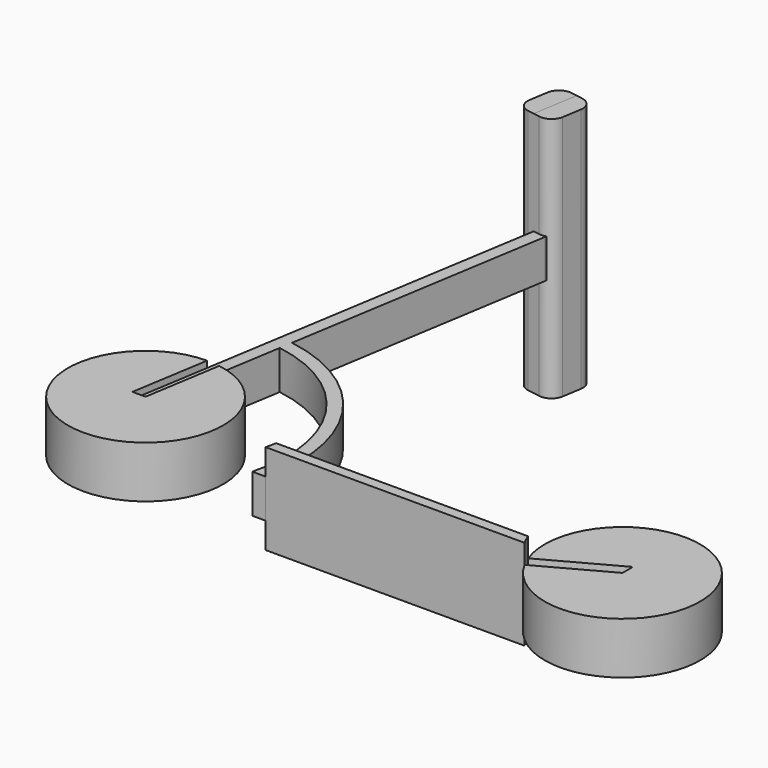
from build123d import *

# Parameters (mm, degrees)
F1_DEPTH      = 50.8
F1_DEPTH_BACK = 50.8
F2_DEPTH      = 38.1
F2_DEPTH_BACK = 38.1
F3_DEPTH      = 88.9
F3_DEPTH_BACK = 88.9
F6_DEPTH      = 88.9
F7_T1_DEPTH   = 609.6
F7_T6_DEPTH   = 609.6
F7_T12_DEPTH  = 609.6
F7_T18_DEPTH  = 609.6
F7_T25_DEPTH  = 609.6
F7_T31_DEPTH  = 609.6


# Not quite as in the source:
# - a fillet or chamfer that OpenCascade refuses, or shapes differently, is made with other operations: its cross-section is extruded or revolved along the edge and cut away or added


with BuildPart() as f1:
    # F0 (on Top) → F1 (new body, two sides)
    with BuildSketch(Plane.XY) as f1_sk:
        with BuildLine():
            ThreePointArc((-783.3901008351, 0), (-819.7667936825, 98.8147367419), (-911.5312057875, 150.4568576405))
            Line((-911.5312057875, 150.4568576405), (-935.7901008351, 0))
            Line((-935.7901008351, 0), (-961.5181404919, 0))
            Line((-961.5181404919, 0), (-936.9466506832, 152.3956114606))
            ThreePointArc((-936.9466506832, 152.3956114606), (-1043.1434934298, -108.1712027225), (-783.3901008351, 0))
        make_face()
    extrude(amount=F1_DEPTH)
    extrude(f1_sk.sketch, amount=-F1_DEPTH_BACK)


with BuildPart() as f1b:
    # F0 (on Top) → F1, piece 2 (new body, two sides)
    with BuildSketch(Plane.XY) as f1_2_sk:
        with BuildLine():
            ThreePointArc((-133.8252661358, -72.9147320071), (37.6217320235, -147.6833276966), (152.4, 0))
            ThreePointArc((152.4, 0), (-26.6841566333, 150.0457123172), (-143.0555877267, -52.5438751919))
            Line((-143.0555877267, -52.5438751919), (0, 25.4))
            Line((0, 25.4), (0, 0))
            Line((0, 0), (-133.8252661358, -72.9147320071))
        make_face()
    extrude(amount=F1_DEPTH)
    extrude(f1_2_sk.sketch, amount=-F1_DEPTH_BACK)


with BuildPart() as f2:
    # F0 (on Top) → F2 (new body, two sides)
    with BuildSketch(Plane.XY) as f2_sk:
        with BuildLine():
            Line((-891.6222432269, 273.9348618882), (-887.5790940523, 299.0110048283))
            Line((-887.5790940523, 299.0110048283), (-804.3877526602, 814.9746455529))
            Line((-804.3877526602, 814.9746455529), (-829.4638956003, 819.0177947275))
            Line((-829.4638956003, 819.0177947275), (-936.9466506832, 152.3956114606))
            ThreePointArc((-936.9466506832, 152.3956114606), (-924.1983244388, 151.9585164444), (-911.5312057875, 150.4568576405))
            Line((-911.5312057875, 150.4568576405), (-891.6222432269, 273.9348618882))
        make_face()
        with BuildLine():
            Line((-935.7901008351, 0), (-911.5312057875, 150.4568576405))
            ThreePointArc((-911.5312057875, 150.4568576405), (-924.1983244388, 151.9585164444), (-936.9466506832, 152.3956114606))
            Line((-936.9466506832, 152.3956114606), (-961.5181404919, 0))
            Line((-961.5181404919, 0), (-935.7901008351, 0))
        make_face()
        with BuildLine():
            ThreePointArc((-641.8252661358, -72.9147320071), (-639.4925118211, -62.7663996731), (-637.5099919387, -52.5438751919))
            ThreePointArc((-637.5099919387, -52.5438751919), (-688.9870787149, 175.5566873001), (-887.5790940523, 299.0110048283))
            Line((-887.5790940523, 299.0110048283), (-891.6222432269, 273.9348618882))
            ThreePointArc((-891.6222432269, 273.9348618882), (-702.5631088402, 150.3205854446), (-668.0690705447, -72.9147320071))
            Line((-668.0690705447, -72.9147320071), (-641.8252661358, -72.9147320071))
        make_face()
    extrude(amount=F2_DEPTH)
    extrude(f2_sk.sketch, amount=-F2_DEPTH_BACK)

    # F5 (on line) → F6 (join)
    with BuildSketch(Plane(origin=(107.6913114103, 667.9156770389, 0), x_dir=(0.9872497221, -0.1591791014, 0), z_dir=(-0.1591791014, -0.9872497221, 0))):
        Polygon((-911.0927623749, 0), (-911.0927623749, 241.3), (-949.192252238, 241.4971602735), (-987.291742101, 241.3), (-987.291742101, 0), (-987.291742101, -241.3), (-949.1927623749, -241.3), (-911.0927623749, -241.3), align=None)
    extrude(amount=-F6_DEPTH)

    # F7: fillet of radius 25.4 on 4 edges, made by hand

    # F7_s2 → F7_t1 (cut)
    with BuildSketch(Plane.XY.offset(-304.8)):
        with BuildLine():
            ThreePointArc((-781.6768920702, 875.6329615621), (-786.1625860927, 894.5486832569), (-802.7098858357, 904.7522536768))
            Line((-802.7098858357, 904.7522536768), (-777.6337428956, 900.7091045022))
            Line((-777.6337428956, 900.7091045022), (-781.6768920702, 875.6329615621))
        make_face()
        with BuildLine():
            ThreePointArc((-827.7850215107, 908.7952404451), (-846.7007432055, 904.3095464227), (-856.9043136254, 887.7622466796))
            Line((-856.9043136254, 887.7622466796), (-852.8611644508, 912.8383896197))
            Line((-852.8611644508, 912.8383896197), (-827.7850215107, 908.7952404451))
        make_face()
        with BuildLine():
            ThreePointArc((-841.9360436219, 821.0287401548), (-858.4833433649, 831.2323105747), (-862.9690373873, 850.1480322695))
            Line((-862.9690373873, 850.1480322695), (-867.0121865619, 825.0718893294))
            Line((-867.0121865619, 825.0718893294), (-841.9360436219, 821.0287401548))
        make_face()
    extrude(amount=F7_T1_DEPTH, mode=Mode.SUBTRACT)


with BuildPart() as f2b:
    # F0 (on Top) → F2, piece 2 (new body, two sides)
    with BuildSketch(Plane.XY) as f2_2_sk:
        with BuildLine():
            Line((0, 25.4), (-143.0555877267, -52.5438751919))
            ThreePointArc((-143.0555877267, -52.5438751919), (-138.8146057184, -62.8988492681), (-133.8252661358, -72.9147320071))
            Line((-133.8252661358, -72.9147320071), (0, 0))
            Line((0, 0), (0, 25.4))
        make_face()
    extrude(amount=F2_DEPTH)
    extrude(f2_2_sk.sketch, amount=-F2_DEPTH_BACK)


with BuildPart() as f3:
    # F0 (on Top) → F3 (new body, two sides)
    with BuildSketch(Plane.XY) as f3_sk:
        with BuildLine():
            ThreePointArc((-133.8252661358, -72.9147320071), (-138.8146057184, -62.8988492681), (-143.0555877267, -52.5438751919))
            Line((-143.0555877267, -52.5438751919), (-637.5099919387, -52.5438751919))
            ThreePointArc((-637.5099919387, -52.5438751919), (-639.4925118211, -62.7663996731), (-641.8252661358, -72.9147320071))
            Line((-641.8252661358, -72.9147320071), (-133.8252661358, -72.9147320071))
        make_face()
    extrude(amount=F3_DEPTH)
    extrude(f3_sk.sketch, amount=-F3_DEPTH_BACK)


with BuildPart() as f7_tool4:
    # F7_s5 → F7_t6 (new body)
    with BuildSketch(Plane.XY.offset(304.8)):
        with BuildLine():
            ThreePointArc((-787.7416158321, 838.0187471519), (-797.945186252, 821.4714474089), (-816.8609079468, 816.9857533865))
            Line((-816.8609079468, 816.9857533865), (-791.7847650068, 812.9426042119))
            Line((-791.7847650068, 812.9426042119), (-787.7416158321, 838.0187471519))
        make_face()
    extrude(amount=-F7_T6_DEPTH)

    split(bisect_by=Plane.XY.offset(38.1), keep=Keep.TOP)

    split(bisect_by=Plane(origin=(-912.0790640705, 147.058968514, 0), x_dir=(0, 0, 1), z_dir=(0.9872497221, -0.1591791014, 0)), keep=Keep.TOP)


with BuildPart() as f2_1:
    add(f2.part)

    # F7_t3: cut F7_tool4
    add(f7_tool4.part, mode=Mode.SUBTRACT)


with BuildPart() as f7_tool10:
    # F7_s11 → F7_t12 (new body)
    with BuildSketch(Plane.XY.offset(304.8)):
        with BuildLine():
            ThreePointArc((-787.7416158321, 838.0187471519), (-797.945186252, 821.4714474089), (-816.8609079468, 816.9857533865))
            Line((-816.8609079468, 816.9857533865), (-791.7847650068, 812.9426042119))
            Line((-791.7847650068, 812.9426042119), (-787.7416158321, 838.0187471519))
        make_face()
    extrude(amount=-F7_T12_DEPTH)

    split(bisect_by=Plane.XY.offset(38.1), keep=Keep.TOP)

    split(bisect_by=Plane(origin=(-912.0790640705, 147.058968514, 0), x_dir=(0, 0, 1), z_dir=(-0.9872497221, 0.1591791014, 0)), keep=Keep.TOP)


with BuildPart() as f2_2:
    add(f2_1.part)

    # F7_t9: cut F7_tool10
    add(f7_tool10.part, mode=Mode.SUBTRACT)


with BuildPart() as f7_tool16:
    # F7_s17 → F7_t18 (new body)
    with BuildSketch(Plane.XY.offset(304.8)):
        with BuildLine():
            ThreePointArc((-787.7416158321, 838.0187471519), (-797.945186252, 821.4714474089), (-816.8609079468, 816.9857533865))
            Line((-816.8609079468, 816.9857533865), (-791.7847650068, 812.9426042119))
            Line((-791.7847650068, 812.9426042119), (-787.7416158321, 838.0187471519))
        make_face()
    extrude(amount=-F7_T18_DEPTH)

    split(bisect_by=Plane.XY.offset(38.1), keep=Keep.BOTTOM)

    split(bisect_by=Plane.XY.offset(-38.1), keep=Keep.TOP)

    split(bisect_by=Plane(origin=(-912.0790640705, 147.058968514, 0), x_dir=(0, 0, 1), z_dir=(0.9872497221, -0.1591791014, 0)), keep=Keep.TOP)


with BuildPart() as f2_3:
    add(f2_2.part)

    # F7_t15: cut F7_tool16
    add(f7_tool16.part, mode=Mode.SUBTRACT)


with BuildPart() as f7_tool23:
    # F7_s24 → F7_t25 (new body)
    with BuildSketch(Plane.XY.offset(304.8)):
        with BuildLine():
            ThreePointArc((-787.7416158321, 838.0187471519), (-797.945186252, 821.4714474089), (-816.8609079468, 816.9857533865))
            Line((-816.8609079468, 816.9857533865), (-791.7847650068, 812.9426042119))
            Line((-791.7847650068, 812.9426042119), (-787.7416158321, 838.0187471519))
        make_face()
    extrude(amount=-F7_T25_DEPTH)

    split(bisect_by=Plane.XY.offset(-38.1), keep=Keep.BOTTOM)

    split(bisect_by=Plane(origin=(-912.0790640705, 147.058968514, 0), x_dir=(0, 0, 1), z_dir=(0.9872497221, -0.1591791014, 0)), keep=Keep.TOP)


with BuildPart() as f2_4:
    add(f2_3.part)

    # F7_t22: cut F7_tool23
    add(f7_tool23.part, mode=Mode.SUBTRACT)


with BuildPart() as f7_tool29:
    # F7_s30 → F7_t31 (new body)
    with BuildSketch(Plane.XY.offset(304.8)):
        with BuildLine():
            ThreePointArc((-787.7416158321, 838.0187471519), (-797.945186252, 821.4714474089), (-816.8609079468, 816.9857533865))
            Line((-816.8609079468, 816.9857533865), (-791.7847650068, 812.9426042119))
            Line((-791.7847650068, 812.9426042119), (-787.7416158321, 838.0187471519))
        make_face()
    extrude(amount=-F7_T31_DEPTH)

    split(bisect_by=Plane.XY.offset(-38.1), keep=Keep.BOTTOM)

    split(bisect_by=Plane(origin=(-912.0790640705, 147.058968514, 0), x_dir=(0, 0, 1), z_dir=(-0.9872497221, 0.1591791014, 0)), keep=Keep.TOP)


with BuildPart() as f2_5:
    add(f2_4.part)

    # F7_t28: cut F7_tool29
    add(f7_tool29.part, mode=Mode.SUBTRACT)


solid = Compound([f1.part, f1b.part, f2b.part, f3.part, f2_5.part])
